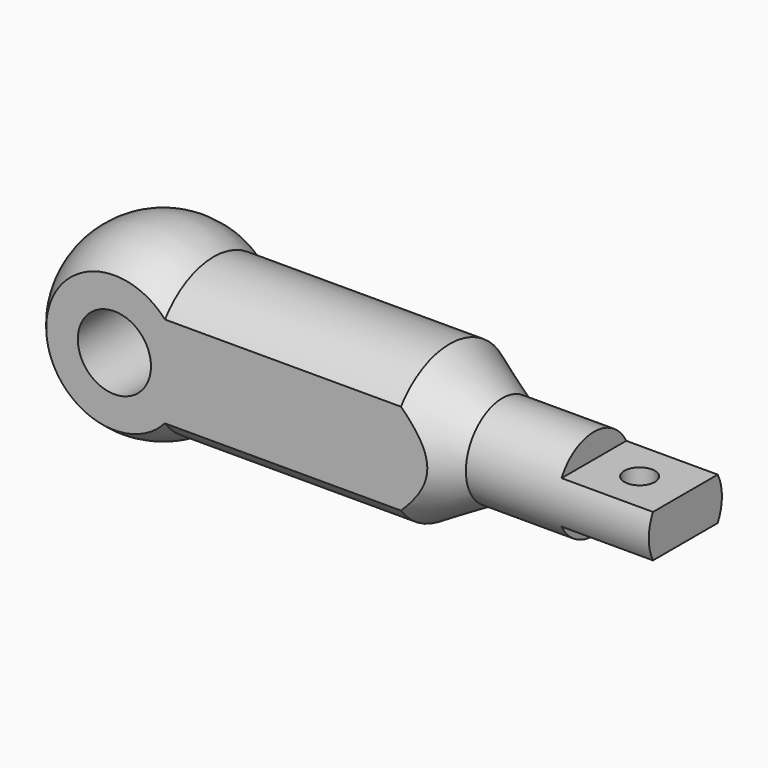
from build123d import *

# Parameters (mm, degrees)
F2_W          = 15
F2_H          = 4
F3_DEPTH      = 15.001
F3_DEPTH_BACK = 15.001
F5_DEPTH      = 100.661254
F6_R          = 6
F7_DEPTH      = 20.001
F8_R          = 2.5
F9_DEPTH      = 18.501


with BuildPart() as f1:
    # F0 (on Front) → F1 (revolve)
    with BuildSketch(Plane.XZ):
        with BuildLine():
            ThreePointArc((8.291562, 12.5), (-7.093186, 13.21691), (-15, 0))
            Line((-15, 0), (85.660254, 0))
            Line((85.660254, 0), (85.660254, 7.5))
            Line((85.660254, 7.5), (55.660254, 7.5))
            Line((55.660254, 7.5), (47, 12.5))
            Line((47, 12.5), (8.291562, 12.5))
        make_face()
    revolve(axis=Axis((50.731633, 0, 0), (1, 0, 0)))

    # F2 (on Front) → F3 (cut, two sides)
    with BuildSketch(Plane.XZ) as f3_sk:
        with Locations((78.160254, 5.5)):
            Rectangle(F2_W, F2_H)
        with Locations((78.160254, -5.5)):
            Rectangle(F2_W, F2_H)
    extrude(amount=-F3_DEPTH, mode=Mode.SUBTRACT)
    extrude(f3_sk.sketch, amount=F3_DEPTH_BACK, mode=Mode.SUBTRACT)

    # F4 (on face) → F5 (cut, through all)
    with BuildSketch(Plane.YZ.offset(85.660254)):
        with BuildLine():
            ThreePointArc((10, -11.18034), (15, 0), (10, 11.18034))
            Line((10, 11.18034), (10, -11.18034))
        make_face()
        with BuildLine():
            Line((-10, -11.18034), (-10, 11.18034))
            ThreePointArc((-10, 11.18034), (-15, 0), (-10, -11.18034))
        make_face()
    extrude(amount=-F5_DEPTH, mode=Mode.SUBTRACT)

    # F6 (on face) → F7 (cut, through all)
    with BuildSketch(Plane.XZ.offset(10)):
        Circle(F6_R)
    extrude(amount=-F7_DEPTH, mode=Mode.SUBTRACT)

    # F8 (on face) → F9 (cut, through all)
    with BuildSketch(Plane.XY.offset(3.5)):
        with Locations((78.160254, 0)):
            Circle(F8_R)
    extrude(amount=-F9_DEPTH, mode=Mode.SUBTRACT)


solid = f1.part
